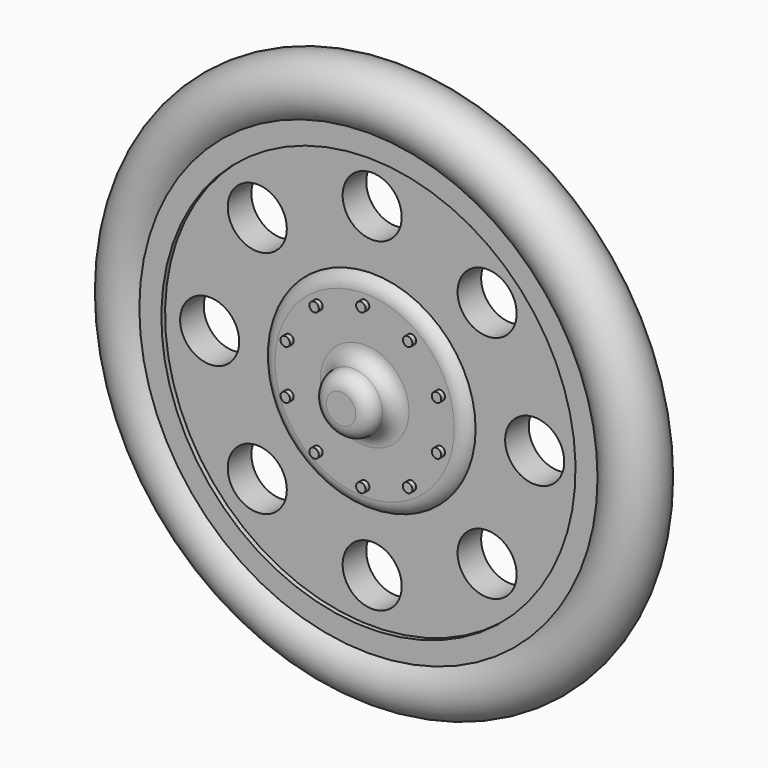
from build123d import *

# Parameters (mm, degrees)
F0_R     = 11.90625
F0_R_2   = 1.5875
F0_R_3   = 5.55625
F1_DEPTH = 1.5875
F2_R     = 5.55625
F3_DEPTH = 0.508
F4_R     = 0.254
F5_DEPTH = 0.254
F6_R     = 1.5875
F7_DEPTH = 1.5875


# Not quite as in the source:
# - a fillet or chamfer that OpenCascade refuses, or shapes differently, is made with other operations: its cross-section is extruded or revolved along the edge and cut away or added


with BuildPart() as f1:
    # F0 (on Front) → F1 (new body)
    with BuildSketch(Plane.XZ):
        Circle(F0_R)
        with Locations((-6.1739260832, -6.1739260832)):
            Circle(F0_R_2, mode=Mode.SUBTRACT)
        with Locations((0, -8.73125)):
            Circle(F0_R_2, mode=Mode.SUBTRACT)
        with Locations((6.1739260832, -6.1739260832)):
            Circle(F0_R_2, mode=Mode.SUBTRACT)
        with Locations((-8.73125, 0)):
            Circle(F0_R_2, mode=Mode.SUBTRACT)
        with Locations((-6.1739260832, 6.1739260832)):
            Circle(F0_R_2, mode=Mode.SUBTRACT)
        Circle(F0_R_3, mode=Mode.SUBTRACT)
        with Locations((8.73125, 0)):
            Circle(F0_R_2, mode=Mode.SUBTRACT)
        with Locations((0, 8.73125)):
            Circle(F0_R_2, mode=Mode.SUBTRACT)
        with Locations((6.1739260832, 6.1739260832)):
            Circle(F0_R_2, mode=Mode.SUBTRACT)
        Circle(F0_R_3)
    extrude(amount=F1_DEPTH)

    # F2 (on face) → F3 (join)
    with BuildSketch(Plane.XZ.offset(1.5875)):
        Circle(F2_R)
    extrude(amount=F3_DEPTH)

    # F4 (on face) → F5 (join)
    with BuildSketch(Plane.XZ.offset(2.0955)):
        with Locations((-2.5119149548, 3.4573543295)):
            Circle(F4_R)
        with Locations((0, 4.2735249735)):
            Circle(F4_R)
        with Locations((2.5119149548, 3.4573543295)):
            Circle(F4_R)
        with Locations((4.0643637736, 1.3205918427)):
            Circle(F4_R)
        with Locations((4.0643637736, -1.3205918427)):
            Circle(F4_R)
        with Locations((2.5119149548, -3.4573543295)):
            Circle(F4_R)
        with Locations((0, -4.2735249735)):
            Circle(F4_R)
        with Locations((-2.5119149548, -3.4573543295)):
            Circle(F4_R)
        with Locations((-4.0643637736, -1.3205918427)):
            Circle(F4_R)
        with Locations((-4.0643637736, 1.3205918427)):
            Circle(F4_R)
    extrude(amount=F5_DEPTH)

    # F6 (on face) → F7 (join)
    with BuildSketch(Plane.XZ.offset(2.0955)):
        Circle(F6_R)
    extrude(amount=F7_DEPTH)

    # F8: fillet of radius 0.79375 on 3 edges, made by hand

    # F8_s1 → F8_t2 (revolve)
    with BuildSketch(Plane.XY):
        with BuildLine():
            ThreePointArc((2.38125, -2.0955), (1.8199839924, -2.3279839924), (1.5875, -2.88925))
            Line((1.5875, -2.88925), (1.5875, -2.0955))
            Line((1.5875, -2.0955), (2.38125, -2.0955))
        make_face()
    revolve(axis=Axis((0, -2.0955, 0), (0, -1, 0)))

    # F8_s3 → F8_t4 (revolve, cut)
    with BuildSketch(Plane.XY):
        with BuildLine():
            ThreePointArc((5.55625, -1.5875), (5.2647319154, -1.9562930181), (4.8157191094, -2.0955))
            Line((4.8157191094, -2.0955), (5.55625, -2.0955))
            Line((5.55625, -2.0955), (5.55625, -1.5875))
        make_face()
    revolve(axis=Axis((0, -2.0955, 0), (0, -1, 0)), mode=Mode.SUBTRACT)

    # F8_s5 → F8_t6 (revolve, cut)
    with BuildSketch(Plane.XY):
        with BuildLine():
            ThreePointArc((1.5875, -2.88925), (1.3550160076, -3.4505160076), (0.79375, -3.683))
            Line((0.79375, -3.683), (1.5875, -3.683))
            Line((1.5875, -3.683), (1.5875, -2.88925))
        make_face()
    revolve(axis=Axis((0, -3.683, 0), (0, -1, 0)), mode=Mode.SUBTRACT)

    # F9 (on Right) → F10 (revolve)
    with BuildSketch(Plane.YZ):
        with BuildLine():
            Line((0.2513255238, 11.1275145485), (0.2513255238, 12.3085637603))
            ThreePointArc((0.2513255238, 12.3085637603), (-0.79375, 15.0910421699), (-1.8388255238, 12.3085637603))
            Line((-1.8388255238, 12.3085637603), (-1.8388255238, 11.1275145485))
            Line((-1.8388255238, 11.1275145485), (0.2513255238, 11.1275145485))
        make_face()
    revolve(axis=Axis((0, -1.3428883394, 0), (0, 1, 0)))


solid = f1.part
